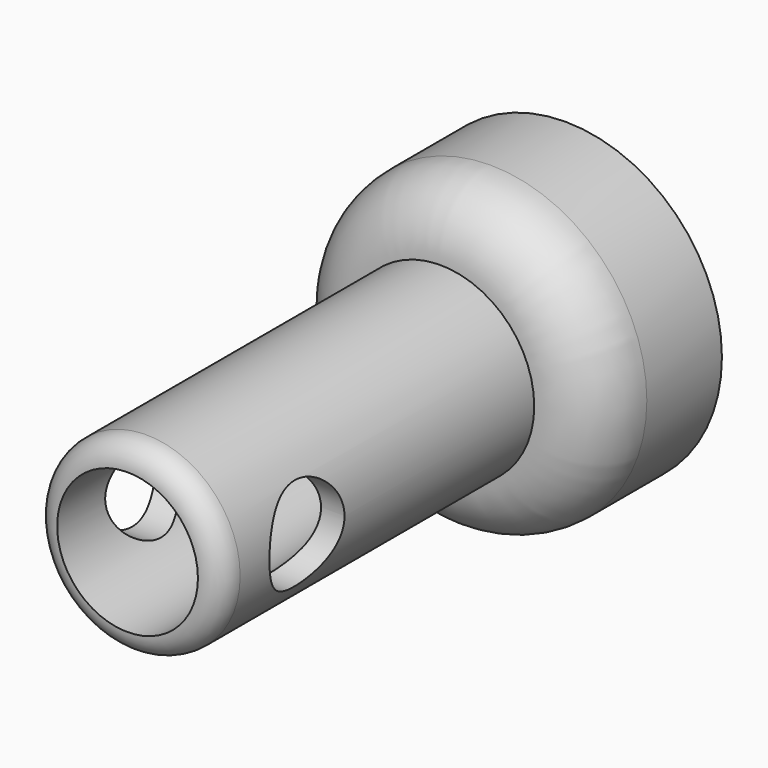
from build123d import *

# Parameters (mm, degrees)
F0_R          = 50.8
F1_DEPTH      = 50.8
F2_R          = 20.32
F3_DEPTH      = 127
F4_R          = 7.62
F5_DEPTH      = 231.902
F6_R          = 15.24
F7_DEPTH      = 114.3
F7_DEPTH_BACK = 213.36


with BuildPart() as f1:
    # F0 (on Front) → F1 (new body)
    with BuildSketch(Plane.XZ):
        with Locations((-16.6321154684, 18.2440392673)):
            Circle(F0_R)
    extrude(amount=F1_DEPTH)

    # F2
    f2_edges = [f1.edges().sort_by_distance(p)[0] for p in [
        (-67.432115, -50.8, 18.244039),
    ]]
    fillet(f2_edges, radius=F2_R)

    # F3 (add): a face of the model
    f3_faces = [f1.faces().sort_by_distance(p)[0] for p in [
        (-16.6321154684, -50.8, 18.2440392673),
    ]]
    extrude(f3_faces, amount=F3_DEPTH)

    # F4
    f4_edges = [f1.edges().sort_by_distance(p)[0] for p in [
        (-47.112115, -177.8, 18.244039),
    ]]
    fillet(f4_edges, radius=F4_R)

    # F5 (cut): a face of the model
    f5_faces = [f1.faces().sort_by_distance(p)[0] for p in [
        (-16.6321154684, -177.8, 18.2440392673),
    ]]
    extrude(f5_faces, amount=-F5_DEPTH, mode=Mode.SUBTRACT)

    # F6 (on Right) → F7 (cut, two sides)
    with BuildSketch(Plane.YZ) as f7_sk:
        with Locations((-143.0514454842, 18.0790871382)):
            Circle(F6_R)
    extrude(amount=F7_DEPTH, mode=Mode.SUBTRACT)
    extrude(f7_sk.sketch, amount=-F7_DEPTH_BACK, mode=Mode.SUBTRACT)


solid = f1.part
